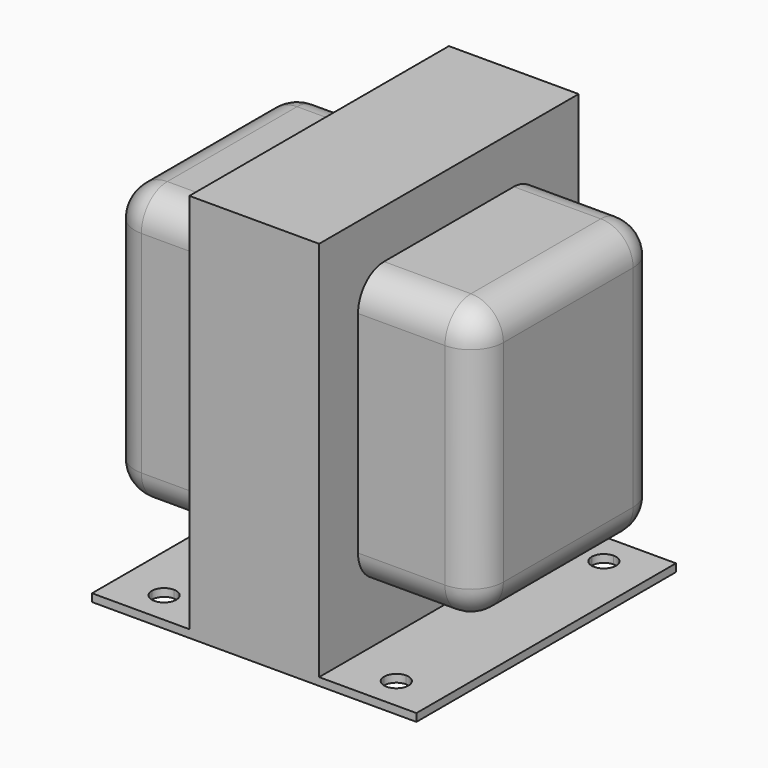
from build123d import *

# Parameters (mm, degrees)
F0_W             = 12.7
F0_H             = 74.676
F0_W_2           = 19.05
F0_H_2           = 1.524
F1_DEPTH         = 31.75
F3_W             = 44.45
F3_H             = 53.975
F4_DEPTH         = 36.068
F6_DEPTH         = 1.524
F6_COPIES2_COUNT = 2
F6_COPIES2_PITCH = 68.174755
F7_R             = 6.35
F8_R             = 6.35


# Not quite as in the source:
# - a pattern or mirror of a feature is missing from the dataset's text; its kind, count and spacing are read off the source's solid


with BuildPart() as f1:
    # F0 (on Front) → F1 (new body, symmetric)
    with BuildSketch(Plane.XZ):
        with Locations((-6.35, 38.862)):
            Rectangle(F0_W, F0_H)
        with Locations((-22.225, 0.762)):
            Rectangle(F0_W_2, F0_H_2)
        with Locations((-6.35, 0.762)):
            Rectangle(F0_W, F0_H_2)
    extrude(amount=F1_DEPTH, both=True)

    # F2: F1 across plane


with BuildPart() as f1_1:
    add(f1.part)
    add(f1.part.mirror(Plane.YZ))

    # F3 (on Right) → F4 (join, symmetric)
    with BuildSketch(Plane.YZ):
        with Locations((0, 39.6875)):
            Rectangle(F3_W, F3_H)
    extrude(amount=F4_DEPTH, both=True)

    # F5 (on face) → F6 (cut, through all)
    with BuildSketch(Plane(origin=(0, 0, 0), x_dir=(1, 0, 0), z_dir=(0, 0, -1))):
        with BuildLine():
            Line((22.72538, 23.0116418839), (22.74062, 23.0116418839))
            ThreePointArc((22.74062, 23.0116418839), (24.4235199971, 23.7087218868), (25.1206, 25.3916218839))
            Line((25.1206, 25.3916218839), (25.1206, 25.4083781161))
            ThreePointArc((25.1206, 25.4083781161), (24.4235199971, 27.0912781132), (22.74062, 27.7883581161))
            Line((22.74062, 27.7883581161), (22.72538, 27.7883581161))
            ThreePointArc((22.72538, 27.7883581161), (21.0424800029, 27.0912781132), (20.3454, 25.4083781161))
            Line((20.3454, 25.4083781161), (20.3454, 25.3916218839))
            ThreePointArc((20.3454, 25.3916218839), (21.0424800029, 23.7087218868), (22.72538, 23.0116418839))
        make_face()
    f6 = extrude(amount=-F6_DEPTH, mode=Mode.SUBTRACT)

    # F6_copies: F6 across plane
    add(f6.mirror(Plane.ZX), mode=Mode.SUBTRACT)

    # F6_copies1: F6 across plane
    add(f6.mirror(Plane(origin=(0, 0, 0), x_dir=(0, 0, -1), z_dir=(-1, 0, 0))), mode=Mode.SUBTRACT)

    # F6_copies2: F6 ×2
    with Locations(*[Vector(-0.666903758, 0.7451438637, 0) * (i * F6_COPIES2_PITCH) for i in range(1, F6_COPIES2_COUNT)]):
        add(f6, mode=Mode.SUBTRACT)

    # F7
    f7_edges = [f1_1.edges().sort_by_distance(p)[0] for p in [
        (24.384, -22.225, 66.675),
        (24.384, 22.225, 66.675),
        (24.384, 22.225, 12.7),
        (24.384, -22.225, 12.7),
        (-24.384, -22.225, 12.7),
        (-24.384, -22.225, 66.675),
        (-24.384, 22.225, 66.675),
        (-24.384, 22.225, 12.7),
    ]]
    fillet(f7_edges, radius=F7_R)

    # F8
    f8_edges = [f1_1.edges().sort_by_distance(p)[0] for p in [
        (-36.068, 22.225, 39.6875),
        (-36.068, 20.365128, 14.559872),
        (-36.068, 20.365128, 64.815128),
        (-36.068, 0, 12.7),
        (-36.068, 0, 66.675),
        (-36.068, -20.365128, 14.559872),
        (-36.068, -20.365128, 64.815128),
        (-36.068, -22.225, 39.6875),
        (36.068, 22.225, 39.6875),
        (36.068, 20.365128, 14.559872),
        (36.068, 20.365128, 64.815128),
        (36.068, 0, 12.7),
        (36.068, 0, 66.675),
        (36.068, -20.365128, 14.559872),
        (36.068, -20.365128, 64.815128),
        (36.068, -22.225, 39.6875),
    ]]
    fillet(f8_edges, radius=F8_R)


solid = f1_1.part
